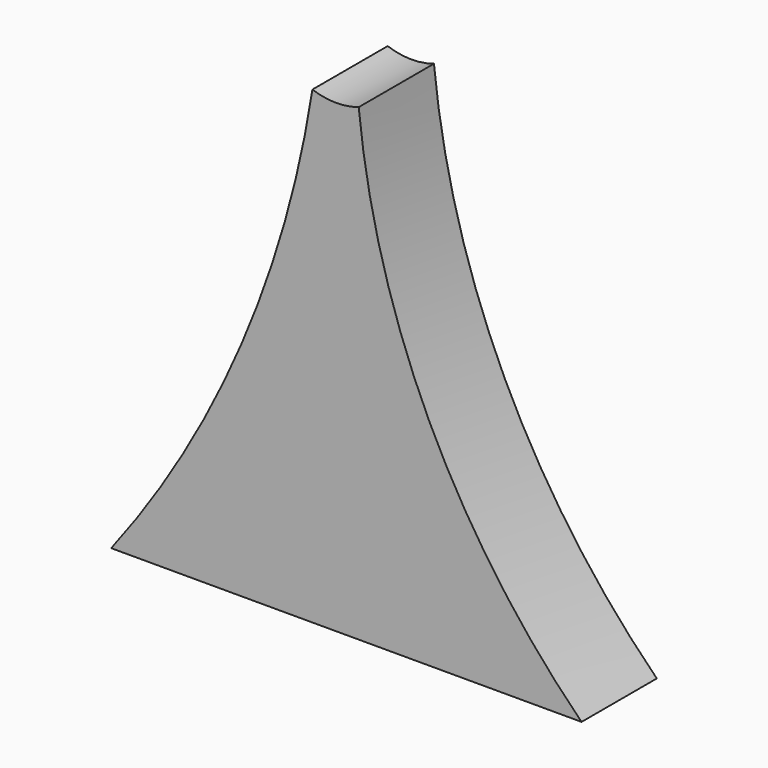
from build123d import *

# Parameters (mm, degrees)
F1_DEPTH = 25.4
F2_DEPTH = 25.4


# Not quite as in the source:
# - a feature names something its author has since deleted; it is built from what else it names


with BuildPart() as f1:
    # F0 (on Front) → F1 (new body)
    with BuildSketch(Plane.XZ):
        with BuildLine():
            ThreePointArc((-18.3465890586, 126.3816356659), (-56.7077419166, -7.1554231915), (-127, -127))
            Line((-127, -127), (127, -127))
            ThreePointArc((127, -127), (44.8039114144, -10.9097348511), (6.6537535749, 126.1220574379))
            ThreePointArc((6.6537535749, 126.1220574379), (-5.8677854381, 124.1938938088), (-18.3465890586, 126.3816356659))
        make_face()
    extrude(amount=F1_DEPTH)

    # F0 (on Front) + F1_face (on face) → F2 (join)
    with BuildSketch(Plane.XZ):
        with BuildLine():
            ThreePointArc((-18.3465890586, 126.3816356659), (-56.7077419166, -7.1554231915), (-127, -127))
            Line((-127, -127), (127, -127))
            ThreePointArc((127, -127), (44.8039114144, -10.9097348511), (6.6537535749, 126.1220574379))
            ThreePointArc((6.6537535749, 126.1220574379), (-5.8677854381, 124.1938938088), (-18.3465890586, 126.3816356659))
        make_face()
    with BuildSketch(Plane(origin=(-4.6947353849, -25.4, -44.0067294457), x_dir=(1, 0, 0), z_dir=(0, -1, 0))):
        with BuildLine():
            ThreePointArc((131.6947353849, -82.9932705543), (49.4986467993, 33.0969945946), (11.3484889598, 170.1287868836))
            ThreePointArc((11.3484889598, 170.1287868836), (-1.1730500532, 168.2006232545), (-13.6518536737, 170.3883651116))
            ThreePointArc((-13.6518536737, 170.3883651116), (-52.0130065317, 36.8513062542), (-122.3052646151, -82.9932705543))
            Line((-122.3052646151, -82.9932705543), (131.6947353849, -82.9932705543))
        make_face()
    extrude(amount=-F2_DEPTH)


solid = f1.part
